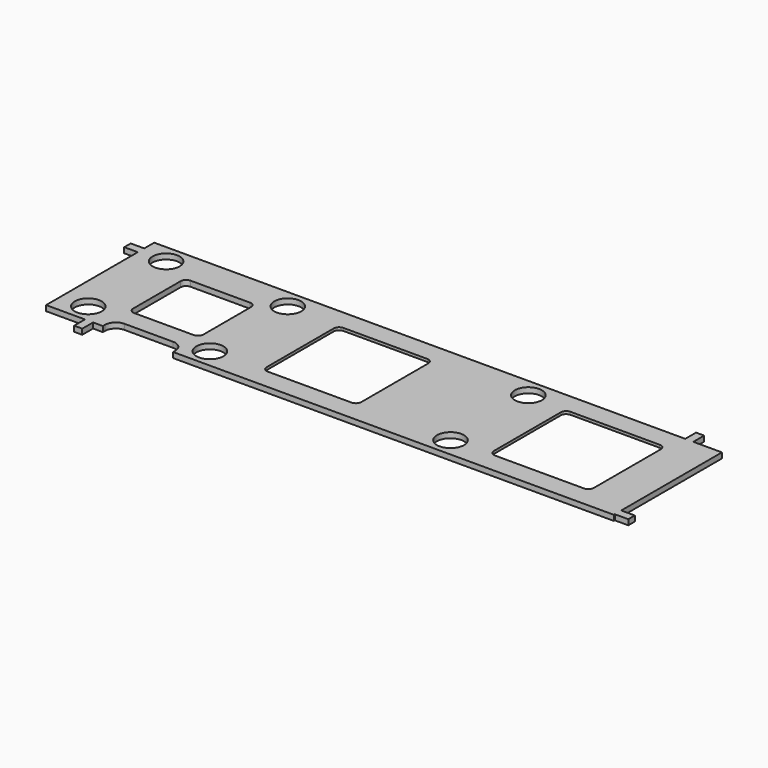
from build123d import *

# Parameters (mm, degrees)
F1_DEPTH  = 2
F2_W      = 26
F2_H      = 26
F3_DEPTH  = 15.4
F4_W      = 35
F4_H      = 35
F4_W_2    = 37
F5_DEPTH  = 25
F6_W      = 26
F6_H      = 5
F7_DEPTH  = 25
F8_R      = 4
F9_R      = 2
F10_R     = 5
F11_DEPTH = 25
F12_R     = 5
F13_DEPTH = 25
F14_W     = 46
F14_H     = 46
F14_W_2   = 48
F15_DEPTH = 1
F16_R     = 1
F17_R     = 1
F0_W      = 5
F0_H      = 3
F0_W_2    = 3
F0_H_2    = 5
F18_DEPTH = 2


# Not quite as in the source:
# - a feature names something its author has since deleted; it is built from what else it names


with BuildPart() as f1:
    # F0 (on Top) → F1 (new body)
    with BuildSketch(Plane.XY):
        Polygon((172.5389735401, 18.1442317292), (-23.8906879723, 18.1442317292), (-23.8906879723, 13.5384923518), (-23.8906879723, 10.5384923518), (-23.8906879723, -31.8557682708), (-9.5117332786, -31.8557682708), (-6.5117332786, -31.8557682708), (186.1093120277, -31.8557682708), (186.1093120277, -31.4002893865), (186.1093120277, -28.4002893865), (186.1093120277, 18.1442317292), (175.5389735401, 18.1442317292), align=None)
    extrude(amount=F1_DEPTH)

    # F2 (on face) → F3 (cut)
    with BuildSketch(Plane(origin=(0, 0, 0), x_dir=(1, 0, 0), z_dir=(0, 0, -1))):
        with Locations((10.1093120277, 6.8557682708)):
            Rectangle(F2_W, F2_H)
    extrude(amount=-F3_DEPTH, mode=Mode.SUBTRACT)

    # F4 (on face) → F5 (cut)
    with BuildSketch(Plane(origin=(0, 0, 0), x_dir=(1, 0, 0), z_dir=(0, 0, -1))):
        with Locations((67.6093120277, 6.8557682708)):
            Rectangle(F4_W, F4_H)
        with Locations((152.6093120277, 6.8557682708)):
            Rectangle(F4_W_2, F4_H)
    extrude(amount=-F5_DEPTH, mode=Mode.SUBTRACT)

    # F6 (on face) → F7 (cut)
    with BuildSketch(Plane.XY.offset(2)):
        with Locations((10.1093120277, -29.3557682708)):
            Rectangle(F6_W, F6_H)
    extrude(amount=-F7_DEPTH, mode=Mode.SUBTRACT)

    # F8
    f8_edges = [f1.edges().sort_by_distance(p)[0] for p in [
        (-2.890688, -26.855768, 1),
        (23.109312, -26.855768, 1),
    ]]
    fillet(f8_edges, radius=F8_R)

    # F9
    f9_edges = [f1.edges().sort_by_distance(p)[0] for p in [
        (50.109312, 10.644232, 1),
        (85.109312, 10.644232, 1),
        (50.109312, -24.355768, 1),
        (134.109312, -24.355768, 1),
        (85.109312, -24.355768, 1),
        (171.109312, -24.355768, 1),
        (134.109312, 10.644232, 1),
        (171.109312, 10.644232, 1),
        (23.109312, 6.144232, 1),
        (-2.890688, 6.144232, 1),
        (23.109312, -19.855768, 1),
        (-2.890688, -19.855768, 1),
    ]]
    fillet(f9_edges, radius=F9_R)

    # F10 (on face) → F11 (cut)
    with BuildSketch(Plane.XY.offset(2)):
        with Locations((120.1093120277, 11.1442317292)):
            Circle(F10_R)
        with Locations((120.1093120277, -24.8557682708)):
            Circle(F10_R)
        with Locations((31.1093120277, -24.8557682708)):
            Circle(F10_R)
        with Locations((-13.8906879723, 11.1442317292)):
            Circle(F10_R)
        with Locations((-13.8906879723, -24.8557682708)):
            Circle(F10_R)
    extrude(amount=-F11_DEPTH, mode=Mode.SUBTRACT)

    # F12 (on face) → F13 (cut)
    with BuildSketch(Plane.XY.offset(2)):
        with Locations((31.1093120277, 11.1442317292)):
            Circle(F12_R)
    extrude(amount=-F13_DEPTH, mode=Mode.SUBTRACT)

    # F14 (on face) → F15 (cut)
    with BuildSketch(Plane.XY):
        with Locations((67.6093120277, -6.8557682708)):
            Rectangle(F14_W, F14_H)
        with Locations((152.6093120277, -6.8557682708)):
            Rectangle(F14_W_2, F14_H)
    extrude(amount=F15_DEPTH, mode=Mode.SUBTRACT)

    # F16
    f16_edges = [f1.edges().sort_by_distance(p)[0] for p in [
        (44.609312, -29.855768, 0.5),
        (90.609312, -29.855768, 0.5),
        (90.609312, 16.144232, 0.5),
        (44.609312, 16.144232, 0.5),
    ]]
    fillet(f16_edges, radius=F16_R)

    # F17
    f17_edges = [f1.edges().sort_by_distance(p)[0] for p in [
        (128.609312, -29.855768, 0.5),
        (176.609312, -29.855768, 0.5),
        (176.609312, 16.144232, 0.5),
        (128.609312, 16.144232, 0.5),
    ]]
    fillet(f17_edges, radius=F17_R)

    # F0 (on Top) → F18 (join)
    with BuildSketch(Plane.XY):
        with Locations((188.6093120277, -29.9002893865)):
            Rectangle(F0_W, F0_H)
        with Locations((174.0389735401, 20.6442317292)):
            Rectangle(F0_W_2, F0_H_2)
        with Locations((-8.0117332786, -34.3557682708)):
            Rectangle(F0_W_2, F0_H_2)
        with Locations((-26.3906879723, 12.0384923518)):
            Rectangle(F0_W, F0_H)
    extrude(amount=F18_DEPTH)


solid = f1.part
